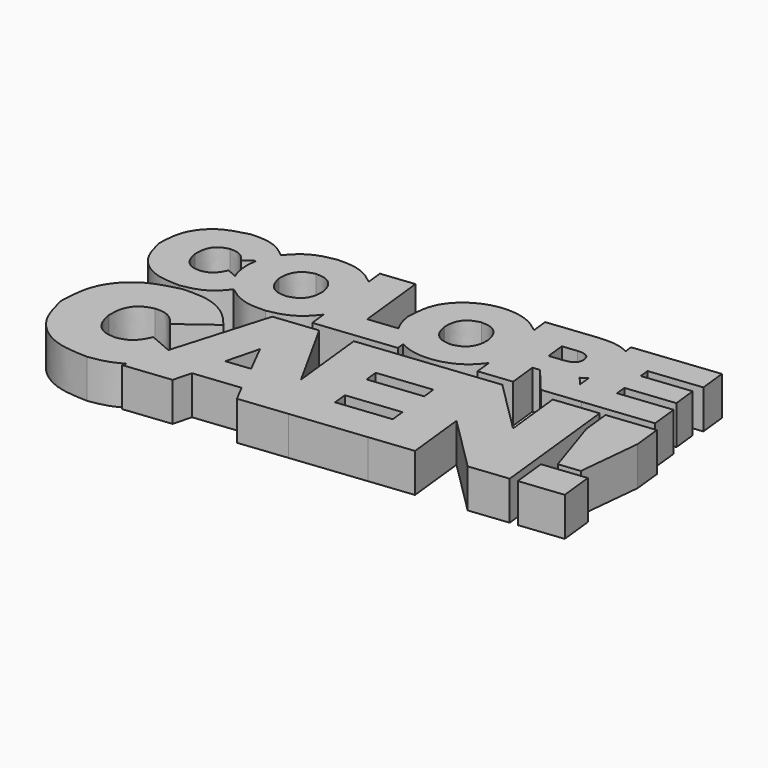
from build123d import *

# Parameters (mm, degrees)
F1_DEPTH = 40
F3_DEPTH = 40


# Not quite as in the source:
# - the dataset's text gives a spline's control points without its knots; the knots are read off the source's solid


with BuildPart() as f1:
    # F0 (on Top) → F1 (new body)
    with BuildSketch(Plane.XY):
        with BuildLine():
            Line((197.7038, 32.87505), (153.1938, 28.00105))
            Line((153.1938, 28.00105), (159.6868, -31.28195))
            Line((159.6868, -31.28195), (105.4228, 22.76905))
            Line((105.4228, 22.76905), (79.1398, 19.89005))
            Line((79.1398, 19.89005), (79.1398, 19.89105))
            Line((79.1398, 19.89105), (-35.3962, 7.34705))
            Line((-35.3962, 7.34705), (-26.7642, -71.46695))
            Line((-26.7642, -71.46695), (-68.8812, 4.65005))
            Line((-68.8812, 4.65005), (-113.3912, -0.22395))
            Line((-113.3912, -0.22395), (-142.2792, -98.02195))
            Line((-142.2792, -98.02195), (-165.8762, -87.90495))
            add(Edge.make_bspline(
                [(-165.8762, -87.90495), (-167.425715, -91.182613), (-170.420573, -97.517586), (-178.52382, -105.29482), (-185.61899, -106.780468), (-189.3512, -107.56195)],
                knots=[0, 0, 0, 0, 10.852529, 20.975454, 32.20987, 32.20987, 32.20987, 32.20987], degree=3))
            add(Edge.make_bspline(
                [(-189.3512, -107.56195), (-194.05005, -107.312475), (-203.459354, -106.812909), (-214.547348, -95.584702), (-216.626282, -85.815893), (-217.7412, -80.57695)],
                knots=[0, 0, 0, 0, 13.712427, 27.458716, 43.35676, 43.35676, 43.35676, 43.35676], degree=3))
            Line((-217.7412, -80.57695), (-217.7832, -80.19295))
            add(Edge.make_bspline(
                [(-217.7832, -80.19295), (-217.777624, -75.08356), (-217.766991, -65.340723), (-209.602702, -52.048893), (-200.461381, -49.412505), (-195.8652, -48.08695)],
                knots=[0, 0, 0, 0, 15.194339, 28.973319, 42.907035, 42.907035, 42.907035, 42.907035], degree=3))
            add(Edge.make_bspline(
                [(-195.8652, -48.08695), (-192.157404, -48.043801), (-185.124188, -47.961952), (-175.811499, -53.544774), (-171.781966, -58.950596), (-169.7132, -61.72595)],
                knots=[0, 0, 0, 0, 10.934971, 20.742249, 31.089715, 31.089715, 31.089715, 31.089715], degree=3))
            Line((-169.7132, -61.72595), (-135.0602, -35.99195))
            add(Edge.make_bspline(
                [(-135.0602, -35.99195), (-140.089083, -30.029476), (-150.264397, -17.965155), (-173.590525, -7.16548), (-190.644331, -7.537407), (-199.7022, -7.73495)],
                knots=[0, 0, 0, 0, 23.223871, 46.990596, 73.913761, 73.913761, 73.913761, 73.913761], degree=3))
            add(Edge.make_bspline(
                [(-199.7022, -7.73495), (-212.097427, -10.880078), (-236.246003, -17.007467), (-261.966724, -47.965593), (-262.916349, -72.847685), (-263.4022, -85.57795)],
                knots=[0, 0, 0, 0, 37.706105, 73.45963, 110.915059, 110.915059, 110.915059, 110.915059], degree=3))
            Line((-263.4022, -85.57795), (-263.3602, -85.96195))
            add(Edge.make_bspline(
                [(-263.3602, -85.96195), (-260.098365, -98.509694), (-253.816708, -122.674193), (-222.338859, -146.760339), (-198.24829, -147.568889), (-186.0902, -147.97695)],
                knots=[0, 0, 0, 0, 38.071591, 73.318435, 109.231698, 109.231698, 109.231698, 109.231698], degree=3))
            add(Edge.make_bspline(
                [(-186.0902, -147.97695), (-181.997056, -147.377589), (-174.201408, -146.236067), (-163.343089, -142.765359), (-157.023271, -139.324995), (-153.9922, -137.67495)],
                knots=[0, 0, 0, 0, 12.399988, 23.616551, 33.954284, 33.954284, 33.954284, 33.954284], degree=3))
            Line((-153.9922, -137.67495), (-155.1742, -141.67895))
            Line((-155.1742, -141.67895), (-107.2112, -136.42595))
            Line((-107.2112, -136.42595), (-102.2802, -117.63495))
            Line((-102.2802, -117.63495), (-55.2762, -112.48795))
            Line((-55.2762, -112.48795), (-46.2022, -129.74395))
            Line((-46.2022, -129.74395), (2.5288, -124.40795))
            Line((2.5288, -124.40795), (2.5288, -124.40695))
            Line((2.5288, -124.40695), (78.1148, -116.12895))
            Line((78.1148, -116.12895), (78.1148, -116.12995))
            Line((78.1148, -116.12995), (122.6248, -111.25495))
            Line((122.6248, -111.25495), (115.8378, -49.28595))
            Line((115.8378, -49.28595), (172.5068, -105.79195))
            Line((172.5068, -105.79195), (212.4118, -101.42195))
            Line((212.4118, -101.42195), (197.7038, 32.87505))
        make_face()
        Polygon((-69.8912, -81.85895), (-94.4482, -84.54795), (-85.7412, -50.58895), align=None, mode=Mode.SUBTRACT)
        Polygon((74.0808, -79.29395), (19.4038, -85.28195), (17.8068, -70.70095), (72.4838, -64.71295), align=None, mode=Mode.SUBTRACT)
        Polygon((14.2558, -38.27795), (12.7648, -24.65595), (67.4408, -18.66795), (68.9328, -32.28995), align=None, mode=Mode.SUBTRACT)
    extrude(amount=F1_DEPTH)


with BuildPart() as f1b:
    # F0 (on Top) → F1, piece 2 (new body)
    with BuildSketch(Plane.XY):
        with BuildLine():
            add(Edge.make_bspline(
                [(-264.5619, 42.24695), (-262.109648, 32.813164), (-257.387076, 14.645484), (-233.721096, -3.463651), (-215.608862, -4.071353), (-206.4679, -4.37805)],
                knots=[0, 0, 0, 0, 28.623364, 55.123159, 82.124192, 82.124192, 82.124192, 82.124192], degree=3))
            add(Edge.make_bspline(
                [(-206.4679, -4.37805), (-200.687092, -3.352657), (-189.991408, -1.45547), (-176.326362, 6.533032), (-170.320141, 14.021442), (-167.4379, 17.61495)],
                knots=[0, 0, 0, 0, 17.522496, 32.420219, 46.165128, 46.165128, 46.165128, 46.165128], degree=3))
            add(Edge.make_bspline(
                [(-167.4379, 17.61495), (-163.428638, 14.68055), (-155.276804, 8.714179), (-140.100245, 4.126862), (-129.541034, 4.467), (-124.1099, 4.64195)],
                knots=[0, 0, 0, 0, 14.836604, 30.166533, 46.40242, 46.40242, 46.40242, 46.40242], degree=3))
            add(Edge.make_bspline(
                [(-124.1099, 4.64195), (-118.54196, 5.713893), (-107.70463, 7.800302), (-93.387443, 16.218361), (-86.668517, 24.386629), (-83.3599, 28.40895)],
                knots=[0, 0, 0, 0, 16.933757, 32.959537, 48.507447, 48.507447, 48.507447, 48.507447], degree=3))
            Line((-83.3599, 28.40895), (-81.5079, 11.49695))
            Line((-81.5079, 11.49695), (-0.2999, 20.39095))
            Line((-0.2999, 20.39095), (-1.1439, 28.09395))
            add(Edge.make_bspline(
                [(-1.1439, 28.09395), (2.23603, 26.525036), (9.10953, 23.334458), (20.623677, 21.280496), (34.200958, 21.409843), (48.914635, 25.153247), (63.257589, 33.326102), (69.973119, 41.526007), (73.2801, 45.56395)],
                knots=[0, 0, 0, 0, 11.140433, 22.655425, 34.727554, 51.66143, 67.68723, 83.235492, 83.235492, 83.235492, 83.235492], degree=3))
            Line((73.2801, 45.56395), (75.1321, 28.65195))
            Line((75.1321, 28.65195), (108.8841, 32.34795))
            Line((108.8841, 32.34795), (105.7251, 61.19695))
            Line((105.7251, 61.19695), (112.6491, 61.95495))
            Line((112.6491, 61.95495), (112.9371, 61.98595))
            Line((112.9371, 61.98595), (135.1361, 35.22295))
            Line((135.1361, 35.22295), (173.6491, 39.44095))
            Line((173.6491, 39.44095), (243.4611, 47.08695))
            Line((243.4611, 47.08695), (240.4281, 74.78095))
            Line((240.4281, 74.78095), (186.7701, 68.90495))
            Line((186.7701, 68.90495), (185.5701, 79.86695))
            Line((185.5701, 79.86695), (234.9001, 85.26995))
            Line((234.9001, 85.26995), (232.2301, 109.64595))
            Line((232.2301, 109.64595), (182.9001, 104.24395))
            Line((182.9001, 104.24395), (181.7781, 114.48495))
            Line((181.7781, 114.48495), (234.7151, 120.28195))
            Line((234.7151, 120.28195), (231.6821, 147.97695))
            Line((231.6821, 147.97695), (145.5701, 138.54595))
            Line((145.5701, 138.54595), (146.4511, 130.50295))
            add(Edge.make_bspline(
                [(146.4511, 130.50295), (143.58999, 131.776279), (137.349553, 134.553569), (125.997201, 135.924424), (117.863467, 135.342173), (113.4041, 135.02295)],
                knots=[0, 0, 0, 0, 9.355168, 20.404784, 33.815062, 33.815062, 33.815062, 33.815062], degree=3))
            Line((113.4041, 135.02295), (64.0741, 129.62095))
            Line((64.0741, 129.62095), (65.8931, 113.00995))
            add(Edge.make_bspline(
                [(65.8931, 113.00995), (61.825293, 116.188741), (53.556494, 122.650401), (37.889953, 127.41431), (17.048532, 128.037121), (-6.851518, 119.361909), (-26.796543, 96.795053), (-27.724368, 77.931376), (-28.1919, 68.42595)],
                knots=[0, 0, 0, 0, 15.378774, 31.261073, 48.101885, 77.336675, 104.741905, 132.57813, 132.57813, 132.57813, 132.57813], degree=3))
            Line((-28.1919, 68.42595), (-28.1609, 68.13695))
            add(Edge.make_bspline(
                [(-28.1609, 68.13695), (-27.781627, 65.645935), (-27.033319, 60.731153), (-24.680719, 53.693411), (-22.380594, 49.412906), (-21.2409, 47.29195)],
                knots=[0, 0, 0, 0, 7.550645, 14.897454, 22.112969, 22.112969, 22.112969, 22.112969], degree=3))
            Line((-21.2409, 47.29195), (-50.9149, 44.04195))
            Line((-50.9149, 44.04195), (-58.8129, 116.16195))
            Line((-58.8129, 116.16195), (-92.5659, 112.46595))
            Line((-92.5659, 112.46595), (-90.7469, 95.85495))
            add(Edge.make_bspline(
                [(-90.7469, 95.85495), (-94.813133, 99.018539), (-103.078811, 105.449359), (-118.76624, 110.457115), (-129.717076, 110.134819), (-135.3529, 109.96895)],
                knots=[0, 0, 0, 0, 15.378321, 31.260441, 48.101204, 48.101204, 48.101204, 48.101204], degree=3))
            add(Edge.make_bspline(
                [(-135.3529, 109.96895), (-140.691951, 108.959245), (-151.089932, 106.992811), (-164.934427, 99.179803), (-171.63836, 91.565628), (-174.9389, 87.81695)],
                knots=[0, 0, 0, 0, 16.23367, 31.615617, 46.532713, 46.532713, 46.532713, 46.532713], degree=3))
            add(Edge.make_bspline(
                [(-174.9389, 87.81695), (-178.573223, 90.783124), (-186.018895, 96.859954), (-200.746858, 101.663062), (-211.180779, 101.268652), (-216.7019, 101.05995)],
                knots=[0, 0, 0, 0, 13.994181, 28.670013, 45.163061, 45.163061, 45.163061, 45.163061], degree=3))
            add(Edge.make_bspline(
                [(-216.7019, 101.05995), (-226.021002, 98.695577), (-244.176708, 94.089247), (-263.514371, 70.814038), (-264.228523, 52.10694), (-264.5939, 42.53595)],
                knots=[0, 0, 0, 0, 28.348357, 55.228977, 83.389125, 83.389125, 83.389125, 83.389125], degree=3))
            Line((-264.5939, 42.53595), (-264.5619, 42.24695))
        make_face()
        with BuildLine():
            add(Edge.make_bspline(
                [(-213.8169, 70.72195), (-211.029425, 70.754497), (-205.741837, 70.816236), (-198.740571, 66.618803), (-195.711192, 62.55455), (-194.1559, 60.46795)],
                knots=[0, 0, 0, 0, 8.220741, 15.594, 23.37344, 23.37344, 23.37344, 23.37344], degree=3))
            Line((-194.1559, 60.46795), (-183.9479, 68.04895))
            add(Edge.make_bspline(
                [(-183.9479, 68.04895), (-184.284009, 66.236661), (-184.961399, 62.584193), (-185.268058, 56.948211), (-184.978295, 53.176501), (-184.8319, 51.27095)],
                knots=[0, 0, 0, 0, 5.52622, 11.137488, 16.867207, 16.867207, 16.867207, 16.867207], degree=3))
            Line((-184.8319, 51.27095), (-184.7999, 50.98295))
            add(Edge.make_bspline(
                [(-184.7999, 50.98295), (-184.564451, 49.286953), (-184.098347, 45.92949), (-182.826629, 41.038583), (-181.625628, 37.934606), (-181.0299, 36.39495)],
                knots=[0, 0, 0, 0, 5.134121, 10.163709, 15.113996, 15.113996, 15.113996, 15.113996], degree=3))
            Line((-181.0299, 36.39495), (-191.2699, 40.78595))
            add(Edge.make_bspline(
                [(-191.2699, 40.78595), (-192.435012, 38.321679), (-194.686897, 33.558828), (-200.779348, 27.711578), (-206.113836, 26.594539), (-208.9199, 26.00695)],
                knots=[0, 0, 0, 0, 8.159515, 15.770406, 24.217034, 24.217034, 24.217034, 24.217034], degree=3))
            add(Edge.make_bspline(
                [(-208.9199, 26.00695), (-212.452672, 26.194672), (-219.526869, 26.570575), (-227.862892, 35.012151), (-229.425765, 42.356393), (-230.2639, 46.29495)],
                knots=[0, 0, 0, 0, 10.309579, 20.644407, 32.596276, 32.596276, 32.596276, 32.596276], degree=3))
            Line((-230.2639, 46.29495), (-230.2959, 46.58395))
            add(Edge.make_bspline(
                [(-230.2959, 46.58395), (-230.291719, 50.425373), (-230.283746, 57.750346), (-224.145303, 67.743446), (-217.272517, 69.725419), (-213.8169, 70.72195)],
                knots=[0, 0, 0, 0, 11.423622, 21.783002, 32.258938, 32.258938, 32.258938, 32.258938], degree=3))
        make_face(mode=Mode.SUBTRACT)
        with BuildLine():
            add(Edge.make_bspline(
                [(-132.3719, 80.07995), (-128.340103, 79.878373), (-120.498933, 79.48634), (-111.385703, 70.870426), (-109.589099, 63.414292), (-108.6729, 59.61195)],
                knots=[0, 0, 0, 0, 11.795848, 22.940952, 34.539178, 34.539178, 34.539178, 34.539178], degree=3))
            Line((-108.6729, 59.61195), (-108.6409, 59.32295))
            add(Edge.make_bspline(
                [(-108.6409, 59.32295), (-108.708085, 55.461824), (-108.839765, 47.894148), (-115.771357, 37.634674), (-123.246161, 35.585326), (-127.0919, 34.53095)],
                knots=[0, 0, 0, 0, 11.452018, 22.445563, 34.095484, 34.095484, 34.095484, 34.095484], degree=3))
            add(Edge.make_bspline(
                [(-127.0919, 34.53095), (-131.12353, 34.732574), (-138.964573, 35.12471), (-148.077853, 43.740427), (-149.874621, 51.196602), (-150.7909, 54.99895)],
                knots=[0, 0, 0, 0, 11.795409, 22.940678, 34.538978, 34.538978, 34.538978, 34.538978], degree=3))
            Line((-150.7909, 54.99895), (-150.8229, 55.28795))
            add(Edge.make_bspline(
                [(-150.8229, 55.28795), (-150.755638, 59.149087), (-150.623806, 66.716818), (-143.692079, 76.976032), (-136.217458, 79.025524), (-132.3719, 80.07995)],
                knots=[0, 0, 0, 0, 11.452044, 22.445717, 34.095227, 34.095227, 34.095227, 34.095227], degree=3))
        make_face(mode=Mode.SUBTRACT)
        with BuildLine():
            add(Edge.make_bspline(
                [(146.3781, 71.19595), (147.101251, 71.664643), (148.533209, 72.592732), (150.562656, 74.117895), (151.822064, 75.221242), (152.4461, 75.76795)],
                knots=[0, 0, 0, 0, 2.584844, 5.11842, 7.606792, 7.606792, 7.606792, 7.606792], degree=3))
            Line((152.4461, 75.76795), (153.9061, 62.42995))
            Line((153.9061, 62.42995), (146.3781, 71.19595))
        make_face(mode=Mode.SUBTRACT)
        with BuildLine():
            add(Edge.make_bspline(
                [(24.2681, 97.23495), (28.29988, 97.033178), (36.140943, 96.64077), (45.254297, 88.025281), (47.050902, 80.569238), (47.9671, 76.76695)],
                knots=[0, 0, 0, 0, 11.795924, 22.940878, 34.538894, 34.538894, 34.538894, 34.538894], degree=3))
            Line((47.9671, 76.76695), (47.9991, 76.47795))
            add(Edge.make_bspline(
                [(47.9991, 76.47795), (47.931955, 72.616666), (47.800357, 65.048884), (40.868596, 54.789424), (33.393835, 52.740245), (29.5481, 51.68595)],
                knots=[0, 0, 0, 0, 11.452459, 22.445822, 34.095659, 34.095659, 34.095659, 34.095659], degree=3))
            add(Edge.make_bspline(
                [(29.5481, 51.68595), (25.516303, 51.887527), (17.675133, 52.27956), (8.561903, 60.895474), (6.765299, 68.351608), (5.8491, 72.15395)],
                knots=[0, 0, 0, 0, 11.795848, 22.940952, 34.539178, 34.539178, 34.539178, 34.539178], degree=3))
            Line((5.8491, 72.15395), (5.8171, 72.44295))
            add(Edge.make_bspline(
                [(5.8171, 72.44295), (5.884285, 76.304076), (6.015965, 83.871752), (12.947557, 94.131226), (20.422361, 96.180574), (24.2681, 97.23495)],
                knots=[0, 0, 0, 0, 11.452018, 22.445563, 34.095484, 34.095484, 34.095484, 34.095484], degree=3))
        make_face(mode=Mode.SUBTRACT)
        with BuildLine():
            add(Edge.make_bspline(
                [(115.6351, 106.65695), (117.943882, 106.781779), (122.09607, 107.006275), (128.043247, 104.067753), (129.031157, 100.30376), (129.5311, 98.39895)],
                knots=[0, 0, 0, 0, 6.913826, 12.434045, 18.089736, 18.089736, 18.089736, 18.089736], degree=3))
            Line((129.5311, 98.39895), (129.5631, 98.10995))
            add(Edge.make_bspline(
                [(129.5631, 98.10995), (129.477362, 96.183963), (129.305206, 92.316727), (124.189269, 88.014246), (119.997189, 87.286524), (117.6551, 86.87995)],
                knots=[0, 0, 0, 0, 5.560172, 11.164403, 18.259358, 18.259358, 18.259358, 18.259358], degree=3))
            Line((117.6551, 86.87995), (103.0871, 85.28495))
            Line((103.0871, 85.28495), (100.9231, 105.04595))
            Line((100.9231, 105.04595), (115.6351, 106.65695))
        make_face(mode=Mode.SUBTRACT)
    extrude(amount=F1_DEPTH)


with BuildPart() as f1c:
    # F0 (on Top) → F1, piece 3 (new body)
    with BuildSketch(Plane.XY):
        Polygon((203.2674, 33.48485), (206.4184, 4.70685), (226.8234, -57.51815), (248.6954, -55.12215), (255.1494, 10.04385), (251.9974, 38.82185), align=None)
    extrude(amount=F1_DEPTH)


with BuildPart() as f1d:
    # F0 (on Top) → F1, piece 4 (new body)
    with BuildSketch(Plane.XY):
        Polygon((264.5939, -95.70705), (260.8129, -61.17305), (216.3019, -66.04805), (220.0849, -100.58105), align=None)
    extrude(amount=F1_DEPTH)


with BuildPart() as f3:
    # F0 (on Top) → F3 (new body)
    with BuildSketch(Plane.XY):
        Polygon((203.2674, 33.48485), (206.4184, 4.70685), (226.8234, -57.51815), (248.6954, -55.12215), (255.1494, 10.04385), (251.9974, 38.82185), align=None)
    extrude(amount=F3_DEPTH)


solid = Compound([f1.part, f1b.part, f1d.part, f3.part])
